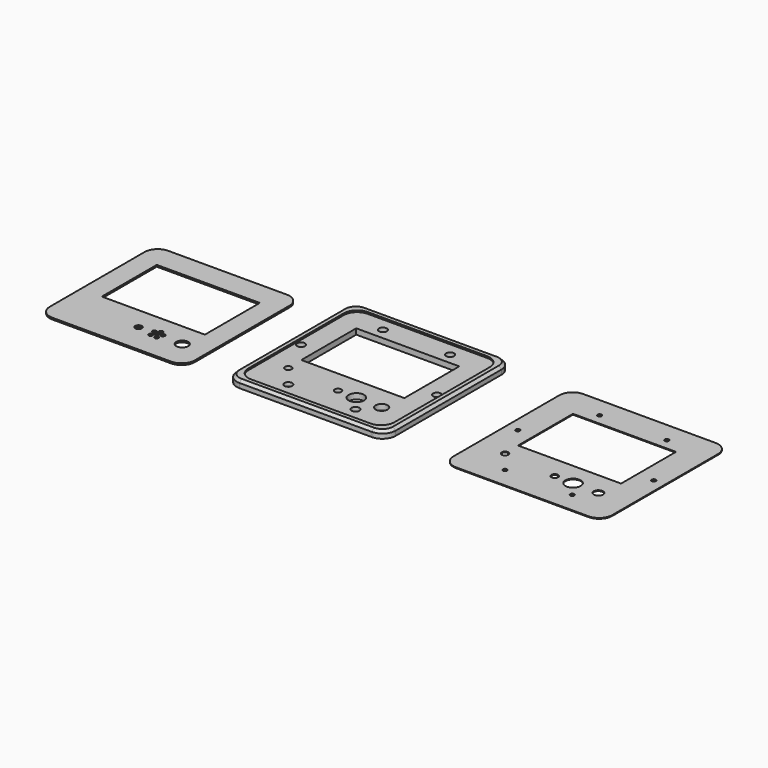
from build123d import *

# Parameters (mm, degrees)
F0_R      = 1.5908867155
F0_R_2    = 2.5705904527
F0_R_3    = 5.9126459129
F0_R_4    = 4.5672278398
F1_DEPTH  = 5.588
F2_R      = 10.16
F3_SIZE   = 2.032
F0_R_5    = 3.556
F4_DEPTH  = 0.635
F5_R      = 10.16
F7_DEPTH  = 1.27
F8_R      = 3.048
F9_DEPTH  = 3.048
F10_R     = 2.5705904527
F10_R_2   = 1.5233915353
F10_R_3   = 4.5672278398
F11_DEPTH = 1.27


# Not quite as in the source:
# - ends of sketch curves that miss each other by under 0.0002 mm in the source are joined


with BuildPart() as f1:
    # F0 (on Top) → F1 (new body)
    with BuildSketch(Plane.XY):
        Polygon((-1.3189034303, 59.5134341434), (-62.4440034303, 59.5134341434), (-62.4440034303, -62.7367658566), (59.8061965697, -62.7367658566), (59.8061965697, 59.5134341434), align=None)
        with Locations((-27.1973789436, -47.042830537)):
            Circle(F0_R, mode=Mode.SUBTRACT)
        with Locations((1.1290358546, -34.6193742007)):
            Circle(F0_R_2, mode=Mode.SUBTRACT)
        with Locations((24.5595706861, -47.042830537)):
            Circle(F0_R, mode=Mode.SUBTRACT)
        with Locations((15.450949059, -34.8733179271)):
            Circle(F0_R_3, mode=Mode.SUBTRACT)
        with Locations((35.3029502789, -35.3193674237)):
            Circle(F0_R_4, mode=Mode.SUBTRACT)
        with Locations((-40.5484696616, -30.3520541638)):
            Circle(F0_R_2, mode=Mode.SUBTRACT)
        with Locations((-53.5016377839, -1.8492421368)):
            Circle(F0_R, mode=Mode.SUBTRACT)
        with Locations((51.1068607298, -1.8492421368)):
            Circle(F0_R, mode=Mode.SUBTRACT)
        Polygon((-40.9749911864, 35.5504732579), (-1.3189034303, 35.5504732579), (38.3371843259, 35.5504732579), (38.3371843259, -17.3154491931), (-40.9749895334, -17.3154491931), align=None, mode=Mode.SUBTRACT)
        with Locations((-27.1973782451, 43.965369463)):
            Circle(F0_R, mode=Mode.SUBTRACT)
        with BuildLine():
            ThreePointArc((26.1504581, 43.965369463), (24.5595713845, 42.3744827475), (22.9686846691, 43.965369463))
            ThreePointArc((22.9686846691, 43.965369463), (24.5595713845, 45.5562561785), (26.1504581, 43.965369463))
        make_face(mode=Mode.SUBTRACT)
    extrude(amount=F1_DEPTH)

    # F2
    f2_edges = [f1.edges().sort_by_distance(p)[0] for p in [
        (-62.444003, 59.513434, 2.794),
        (-62.444003, -62.736766, 2.794),
        (59.806197, -62.736766, 2.794),
        (59.806197, 59.513434, 2.794),
    ]]
    fillet(f2_edges, radius=F2_R)

    # F3
    f3_edges = [f1.edges().sort_by_distance(p)[0] for p in [
        (-1.318903, 59.513434, 5.588),
    ]]
    chamfer(f3_edges, length=F3_SIZE)

    # F6 (on face) → F7 (cut)
    with BuildSketch(Plane.XY.offset(5.588)):
        with BuildLine():
            ThreePointArc((-57.5114712119, -47.565764811), (-54.5356761088, -54.7499697079), (-47.3514712119, -57.725764811))
            Line((-47.3514712119, -57.725764811), (-5.00380015, -57.725764811))
            Line((-5.00380015, -57.725764811), (44.6580416226, -57.725764811))
            ThreePointArc((44.6580416226, -57.725764811), (51.8422465195, -54.7499697079), (54.8180416226, -47.565764811))
            Line((54.8180416226, -47.565764811), (54.8180416226, 0))
            Line((54.8180416226, 0), (54.8180416226, 44.3454599643))
            ThreePointArc((54.8180416226, 44.3454599643), (51.8422465195, 51.5296648611), (44.6580416226, 54.5054599643))
            Line((44.6580416226, 54.5054599643), (-1.3284197776, 54.5054599643))
            Line((-1.3284197776, 54.5054599643), (-47.3514712119, 54.5054599643))
            ThreePointArc((-47.3514712119, 54.5054599643), (-54.5356761088, 51.5296648611), (-57.5114712119, 44.3454599643))
            Line((-57.5114712119, 44.3454599643), (-57.5114712119, 0))
            Line((-57.5114712119, 0), (-57.5114712119, -47.565764811))
        make_face()
    extrude(amount=-F7_DEPTH, mode=Mode.SUBTRACT)

    # F8 (on face) → F9 (cut)
    with BuildSketch(Plane.XY.offset(4.318)):
        with Locations((-27.1973782451, 43.965369463)):
            Circle(F8_R)
        with Locations((24.5595713845, 43.965369463)):
            Circle(F8_R)
        with Locations((-27.1973789436, -47.042830537)):
            Circle(F8_R)
        with Locations((24.5595706861, -47.042830537)):
            Circle(F8_R)
        with Locations((-53.5016377839, -1.8492421368)):
            Circle(F8_R)
        with Locations((51.1068607298, -1.8492421368)):
            Circle(F8_R)
    extrude(amount=-F9_DEPTH, mode=Mode.SUBTRACT)


with BuildPart() as f4:
    # F0 (on Top) → F4 (new body)
    with BuildSketch(Plane.XY):
        Polygon((165.490322156, 59.5134341434), (104.365222156, 59.5134341434), (104.365222156, -62.7367658566), (226.615422156, -62.7367658566), (226.615422156, 59.5134341434), align=None)
        with Locations((139.6118466427, -47.042830537)):
            Circle(F0_R, mode=Mode.SUBTRACT)
        with Locations((167.9382614409, -34.6193742007)):
            Circle(F0_R_2, mode=Mode.SUBTRACT)
        with Locations((182.2601746453, -34.8733179271)):
            Circle(F0_R_3, mode=Mode.SUBTRACT)
        with Locations((191.3687962724, -47.042830537)):
            Circle(F0_R, mode=Mode.SUBTRACT)
        with Locations((202.1121758653, -35.3193674237)):
            Circle(F0_R_5, mode=Mode.SUBTRACT)
        with Locations((126.2607559247, -30.3520541638)):
            Circle(F0_R_2, mode=Mode.SUBTRACT)
        with Locations((113.3075878024, -1.8492421368)):
            Circle(F0_R, mode=Mode.SUBTRACT)
        with Locations((217.9160863161, -1.8492421368)):
            Circle(F0_R, mode=Mode.SUBTRACT)
        Polygon((125.8342343999, 35.5504732579), (165.490322156, 35.5504732579), (205.1464099122, 35.5504732579), (205.1464099122, -17.3154491931), (125.8342266083, -17.3154491931), align=None, mode=Mode.SUBTRACT)
        with Locations((139.6118473412, 43.965369463)):
            Circle(F0_R, mode=Mode.SUBTRACT)
        with BuildLine():
            ThreePointArc((192.9596836864, 43.965369463), (191.3687969709, 42.3744827475), (189.7779102554, 43.965369463))
            ThreePointArc((189.7779102554, 43.965369463), (191.3687969709, 45.5562561785), (192.9596836864, 43.965369463))
        make_face(mode=Mode.SUBTRACT)
    extrude(amount=F4_DEPTH)

    # F5
    f5_edges = [f4.edges().sort_by_distance(p)[0] for p in [
        (104.365222, -62.736766, 0.3175),
        (226.615422, -62.736766, 0.3175),
        (104.365222, 59.513434, 0.3175),
        (226.615422, 59.513434, 0.3175),
    ]]
    fillet(f5_edges, radius=F5_R)


with BuildPart() as f11:
    # F10 (on Top) → F11 (new body)
    with BuildSketch(Plane.XY):
        with BuildLine():
            Line((-104.529616534, 48.298209825), (-150.186116534, 48.298209825))
            Line((-150.186116534, 48.298209825), (-195.842616534, 48.298209825))
            ThreePointArc((-195.842616534, 48.298209825), (-203.0268214309, 45.3224148025), (-206.002616534, 38.1382099056))
            Line((-206.002616534, 38.1382099056), (-206.0026116043, -53.0477900944))
            ThreePointArc((-206.0026116043, -53.0477900944), (-203.0268214309, -60.2319949912), (-195.842616534, -63.2077900944))
            Line((-195.842616534, -63.2077900944), (-104.529616534, -63.2077900944))
            ThreePointArc((-104.529616534, -63.2077900944), (-97.3454116372, -60.2319949912), (-94.369616534, -53.0477900944))
            Line((-94.369616534, -53.0477900944), (-94.369616534, 38.1382099056))
            ThreePointArc((-94.369616534, 38.1382099056), (-97.3454116372, 45.3224148025), (-104.529616534, 48.298209825))
        make_face()
        with Locations((-147.7381789022, -40.4640119523)):
            Circle(F10_R, mode=Mode.SUBTRACT)
        with Locations((-136.8286990857, -38.954846561)):
            Circle(F10_R_2, mode=Mode.SUBTRACT)
        with Locations((-135.7924354748, -43.6562315569)):
            Circle(F10_R_2, mode=Mode.SUBTRACT)
        with Locations((-131.0233575588, -43.9531244338)):
            Circle(F10_R_2, mode=Mode.SUBTRACT)
        with Locations((-133.4162640448, -40.7179556787)):
            Circle(F10_R_2, mode=Mode.SUBTRACT)
        with Locations((-129.6917208767, -39.4892096519)):
            Circle(F10_R_2, mode=Mode.SUBTRACT)
        with Locations((-133.3061456046, -36.9704924524)):
            Circle(F10_R_2, mode=Mode.SUBTRACT)
        with Locations((-113.5591906324, -41.1639977247)):
            Circle(F10_R_3, mode=Mode.SUBTRACT)
        Polygon((-189.8422042902, -23.1600869447), (-189.8422042902, 29.7058355063), (-150.186116534, 29.7058355063), (-110.5300287779, 29.7058355063), (-110.5300287779, -23.1600869447), align=None, mode=Mode.SUBTRACT)
    extrude(amount=F11_DEPTH)


solid = Compound([f1.part, f4.part, f11.part])
